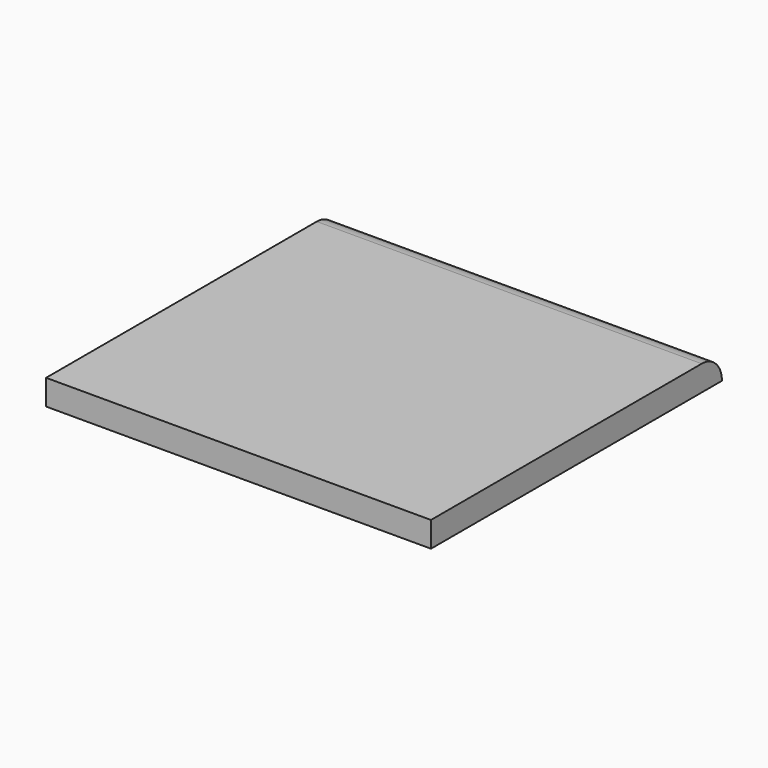
from build123d import *

# Parameters (mm, degrees)
F0_W     = 192.9788589478
F0_H     = 182.3403686285
F1_DEPTH = 12.7
F4_R     = 12.69999


# Not quite as in the source:
# - a fillet or chamfer is up to 0.001 mm smaller than in the source, because OpenCascade refuses the exact size
# - the program builds the solid bodies; features that only make, move or delete a surface that nothing else refers to are left out


with BuildPart() as f1:
    # F0 (on Top) → F1 (new body)
    with BuildSketch(Plane.XY):
        Rectangle(F0_W, F0_H)
    extrude(amount=F1_DEPTH)

    # F4 (radius 12.7 in the source; OpenCascade refuses exactly that, so slightly less here)
    f4_edges = [f1.edges().sort_by_distance(p)[0] for p in [
        (0, 91.170184, 12.7),
    ]]
    fillet(f4_edges, radius=F4_R)


solid = f1.part
